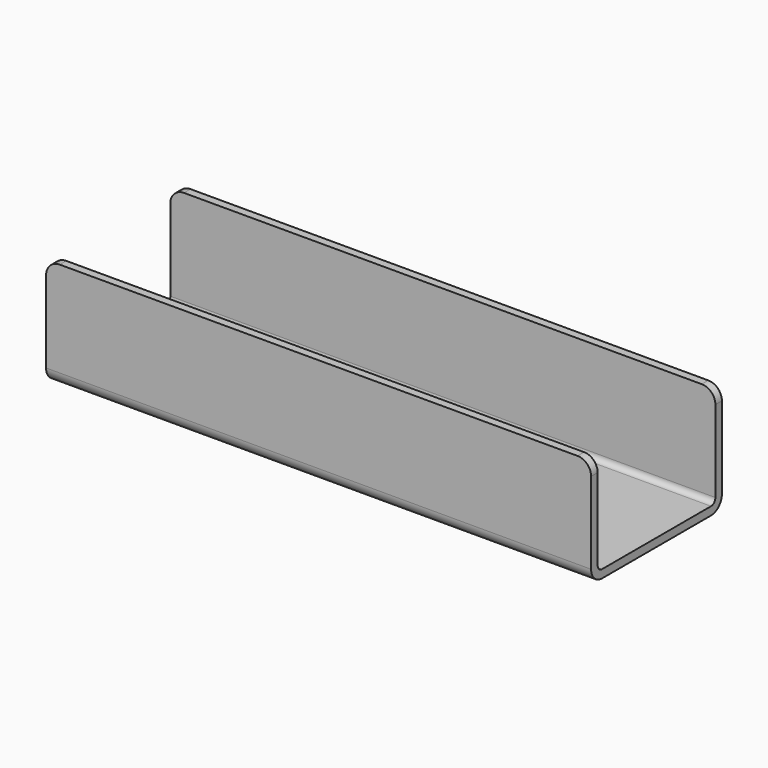
from build123d import *

# Parameters (mm, degrees)
F0_W     = 60
F0_H     = 40
F1_DEPTH = 100
F2_R     = 5
F3_T     = -3
F4_R     = 5


with BuildPart() as f1:
    # F0 (on Right) → F1 (new body, symmetric)
    with BuildSketch(Plane.YZ):
        Rectangle(F0_W, F0_H)
    extrude(amount=F1_DEPTH, both=True)

    # F2
    f2_edges = [f1.edges().sort_by_distance(p)[0] for p in [
        (0, -30, -20),
        (0, 30, -20),
    ]]
    fillet(f2_edges, radius=F2_R)

    # F3
    f3_openings = [f1.faces().sort_by_distance(p)[0] for p in [
        (0, 0, 20),
        (100, 0, 0.084803),
        (-100, 0, 0.084803),
    ]]
    offset(amount=F3_T, openings=f3_openings)

    # F4
    f4_edges = [f1.edges().sort_by_distance(p)[0] for p in [
        (-100, 28.5, 20),
        (-100, -28.5, 20),
        (100, 28.5, 20),
        (100, -28.5, 20),
    ]]
    fillet(f4_edges, radius=F4_R)


solid = f1.part
